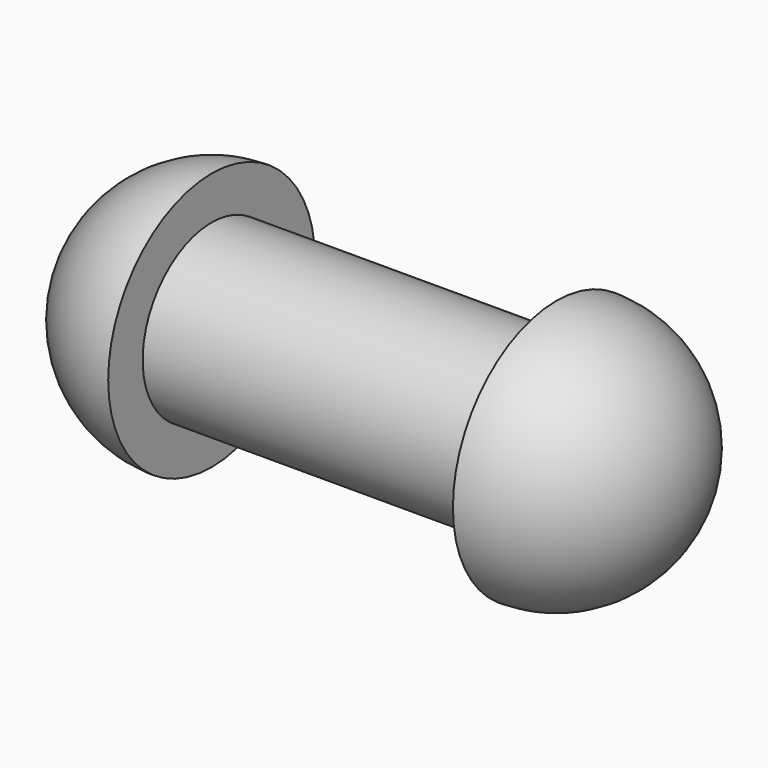
from build123d import *

# Parameters (mm, degrees)
F0_R     = 1
F1_DEPTH = 2
F3_ANGLE = 180


# Not quite as in the source:
# - a pattern or mirror of a feature is missing from the dataset's text; its kind, count and spacing are read off the source's solid


with BuildPart() as f1:
    # F0 (on Right) → F1 (new body, symmetric)
    with BuildSketch(Plane.YZ):
        Circle(F0_R)
    extrude(amount=F1_DEPTH, both=True)

    # F2 (on face) → F3 (revolve)
    with BuildSketch(Plane.YZ.offset(2)):
        with BuildLine():
            Line((0, -1.5), (0, 1.5))
            ThreePointArc((0, 1.5), (-1.5, 0), (0, -1.5))
        make_face()
    f3 = revolve(axis=Axis((2, 0, 0), (0, 0, 1)), revolution_arc=F3_ANGLE)

    # F3_copies: F3 across plane
    add(f3.mirror(Plane(origin=(0, 0, 0), x_dir=(0, 0, -1), z_dir=(-1, 0, 0))))


solid = f1.part
